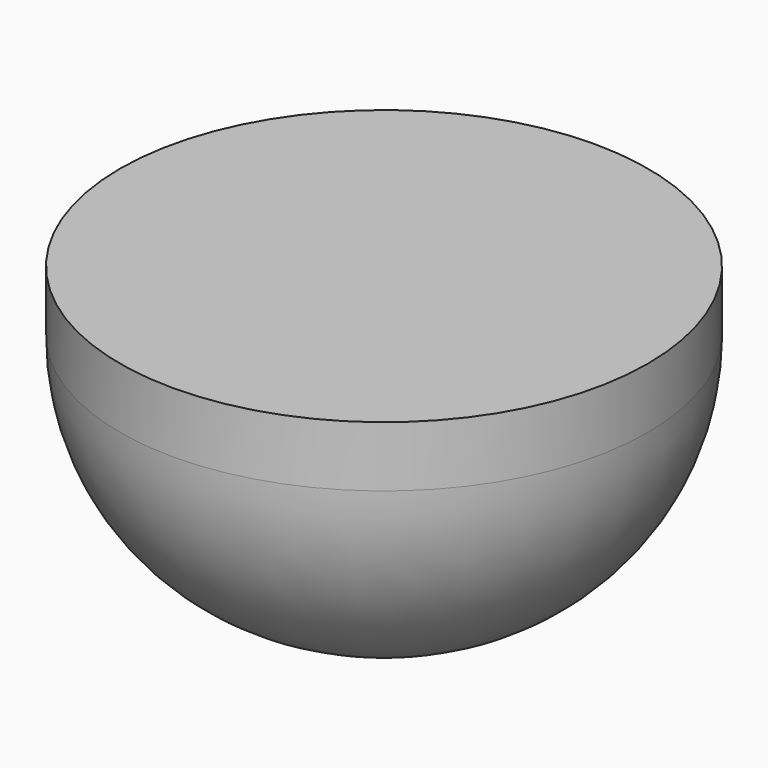
from build123d import *

# Parameters (mm, degrees)
F2_R     = 22.1449066967
F3_DEPTH = 25.4
F4_R     = 20.32


# Not quite as in the source:
# - the program builds the solid bodies; features that only make, move or delete a surface that nothing else refers to are left out


with BuildPart() as f3:
    # F2 (on Top) → F3 (new body)
    with BuildSketch(Plane.XY):
        Circle(F2_R)
    extrude(amount=-F3_DEPTH)

    # F4
    f4_edges = [f3.edges().sort_by_distance(p)[0] for p in [
        (-22.144907, 0, -25.4),
    ]]
    fillet(f4_edges, radius=F4_R)


solid = f3.part
